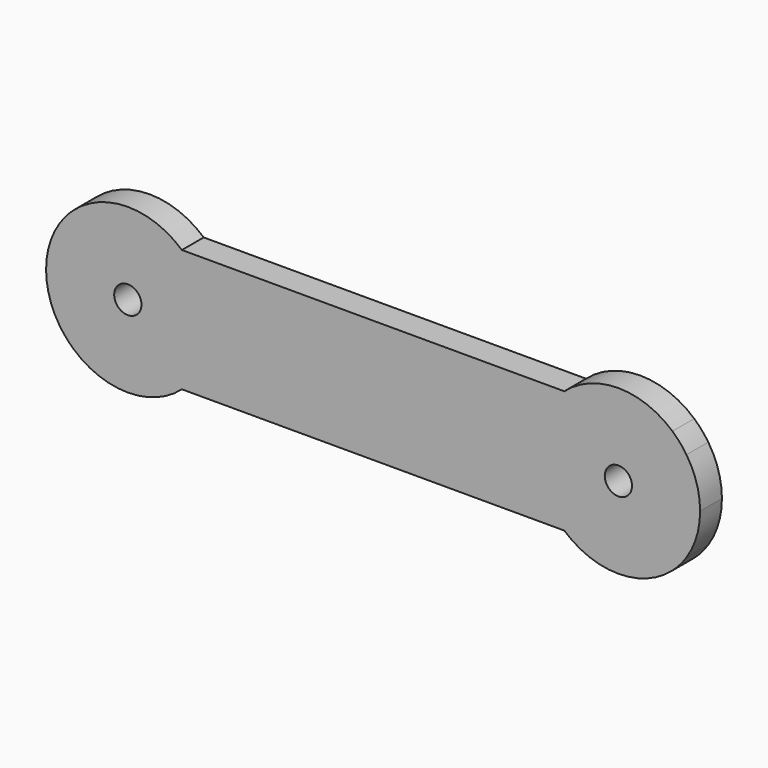
from build123d import *

# Parameters (mm, degrees)
F0_R     = 1
F1_DEPTH = 2


with BuildPart() as f1:
    # F0 (on Front) → F1 (new body)
    with BuildSketch(Plane.XZ):
        with BuildLine():
            ThreePointArc((-49.9391267766, 34.7456367077), (-53.9077537432, 36.2456367077), (-57.8763807098, 34.7456367077))
            Line((-57.8763807098, 34.7456367077), (-49.9391267766, 34.7456367077))
        make_face()
        with BuildLine():
            Line((-49.9391267766, 34.7456367077), (-57.8763807098, 34.7456367077))
            ThreePointArc((-57.8763807098, 34.7456367077), (-58.4309342214, 34.1878237101), (-58.9077537432, 33.562261498))
            Line((-58.9077537432, 33.562261498), (-58.9077537432, 26.9290119173))
            ThreePointArc((-58.9077537432, 26.9290119173), (-58.4309342214, 26.3034497053), (-57.8763807098, 25.7456367077))
            Line((-57.8763807098, 25.7456367077), (-49.9391267766, 25.7456367077))
            ThreePointArc((-49.9391267766, 25.7456367077), (-49.3845732651, 26.3034497053), (-48.9077537432, 26.9290119173))
            Line((-48.9077537432, 26.9290119173), (-48.9077537432, 30.2456367077))
            Line((-48.9077537432, 30.2456367077), (-48.9077537432, 33.562261498))
            ThreePointArc((-48.9077537432, 33.562261498), (-49.3845732651, 34.1878237101), (-49.9391267766, 34.7456367077))
        make_face()
        with Locations((-53.9077537432, 30.2456367077)):
            Circle(F0_R, mode=Mode.SUBTRACT)
        with BuildLine():
            Line((-58.9077537432, 26.9290119173), (-58.9077537432, 33.562261498))
            ThreePointArc((-58.9077537432, 33.562261498), (-59.9077537432, 30.2456367077), (-58.9077537432, 26.9290119173))
        make_face()
        with BuildLine():
            Line((-48.9077537432, 34.7456367077), (-49.9391267766, 34.7456367077))
            ThreePointArc((-49.9391267766, 34.7456367077), (-49.3845732651, 34.1878237101), (-48.9077537432, 33.562261498))
            Line((-48.9077537432, 33.562261498), (-48.9077537432, 34.7456367077))
        make_face()
        with BuildLine():
            Line((-22.9077537432, 34.7456367077), (-48.9077537432, 34.7456367077))
            Line((-48.9077537432, 34.7456367077), (-48.9077537432, 33.562261498))
            ThreePointArc((-48.9077537432, 33.562261498), (-48.1631910967, 31.9776875152), (-47.9077537432, 30.2456367077))
            ThreePointArc((-47.9077537432, 30.2456367077), (-48.1631910967, 28.5135859001), (-48.9077537432, 26.9290119173))
            Line((-48.9077537432, 26.9290119173), (-48.9077537432, 25.7456367077))
            Line((-48.9077537432, 25.7456367077), (-22.9077537432, 25.7456367077))
            Line((-22.9077537432, 25.7456367077), (-22.9077537432, 26.9290119173))
            ThreePointArc((-22.9077537432, 26.9290119173), (-23.9077537432, 30.2456367077), (-22.9077537432, 33.562261498))
            Line((-22.9077537432, 33.562261498), (-22.9077537432, 34.7456367077))
        make_face()
        with BuildLine():
            ThreePointArc((-47.9077537432, 30.2456367077), (-48.1631910967, 31.9776875152), (-48.9077537432, 33.562261498))
            Line((-48.9077537432, 33.562261498), (-48.9077537432, 30.2456367077))
            Line((-48.9077537432, 30.2456367077), (-48.9077537432, 26.9290119173))
            ThreePointArc((-48.9077537432, 26.9290119173), (-48.1631910967, 28.5135859001), (-47.9077537432, 30.2456367077))
        make_face()
        with BuildLine():
            Line((-49.9391267766, 25.7456367077), (-57.8763807098, 25.7456367077))
            ThreePointArc((-57.8763807098, 25.7456367077), (-53.9077537432, 24.2456367077), (-49.9391267766, 25.7456367077))
        make_face()
        with BuildLine():
            Line((-21.8763807098, 34.7456367077), (-22.9077537432, 34.7456367077))
            Line((-22.9077537432, 34.7456367077), (-22.9077537432, 33.562261498))
            ThreePointArc((-22.9077537432, 33.562261498), (-22.4309342214, 34.1878237101), (-21.8763807098, 34.7456367077))
        make_face()
        with BuildLine():
            ThreePointArc((-48.9077537432, 26.9290119173), (-49.3845732651, 26.3034497053), (-49.9391267766, 25.7456367077))
            Line((-49.9391267766, 25.7456367077), (-48.9077537432, 25.7456367077))
            Line((-48.9077537432, 25.7456367077), (-48.9077537432, 26.9290119173))
        make_face()
        with BuildLine():
            ThreePointArc((-13.9391267766, 34.7456367077), (-17.9077537432, 36.2456367077), (-21.8763807098, 34.7456367077))
            Line((-21.8763807098, 34.7456367077), (-13.9391267766, 34.7456367077))
        make_face()
        with BuildLine():
            Line((-13.9391267766, 34.7456367077), (-21.8763807098, 34.7456367077))
            ThreePointArc((-21.8763807098, 34.7456367077), (-22.4309342214, 34.1878237101), (-22.9077537432, 33.562261498))
            Line((-22.9077537432, 33.562261498), (-22.9077537432, 30.2456367077))
            Line((-22.9077537432, 30.2456367077), (-22.9077537432, 26.9290119173))
            ThreePointArc((-22.9077537432, 26.9290119173), (-22.4309342214, 26.3034497053), (-21.8763807098, 25.7456367077))
            Line((-21.8763807098, 25.7456367077), (-13.9391267766, 25.7456367077))
            ThreePointArc((-13.9391267766, 25.7456367077), (-13.3845732651, 26.3034497053), (-12.9077537432, 26.9290119173))
            Line((-12.9077537432, 26.9290119173), (-12.9077537432, 33.562261498))
            ThreePointArc((-12.9077537432, 33.562261498), (-13.3845732651, 34.1878237101), (-13.9391267766, 34.7456367077))
        make_face()
        with BuildLine():
            ThreePointArc((-16.9077537432, 30.2456367077), (-17.9077537432, 29.2456367077), (-18.9077537432, 30.2456367077))
            ThreePointArc((-18.9077537432, 30.2456367077), (-17.9077537432, 31.2456367077), (-16.9077537432, 30.2456367077))
        make_face(mode=Mode.SUBTRACT)
        with BuildLine():
            Line((-22.9077537432, 30.2456367077), (-22.9077537432, 33.562261498))
            ThreePointArc((-22.9077537432, 33.562261498), (-23.9077537432, 30.2456367077), (-22.9077537432, 26.9290119173))
            Line((-22.9077537432, 26.9290119173), (-22.9077537432, 30.2456367077))
        make_face()
        with BuildLine():
            ThreePointArc((-21.8763807098, 25.7456367077), (-22.4309342214, 26.3034497053), (-22.9077537432, 26.9290119173))
            Line((-22.9077537432, 26.9290119173), (-22.9077537432, 25.7456367077))
            Line((-22.9077537432, 25.7456367077), (-21.8763807098, 25.7456367077))
        make_face()
        with BuildLine():
            ThreePointArc((-11.9077537432, 30.2456367077), (-12.1631910967, 31.9776875152), (-12.9077537432, 33.562261498))
            Line((-12.9077537432, 33.562261498), (-12.9077537432, 26.9290119173))
            ThreePointArc((-12.9077537432, 26.9290119173), (-12.1631910967, 28.5135859001), (-11.9077537432, 30.2456367077))
        make_face()
        with BuildLine():
            Line((-13.9391267766, 25.7456367077), (-21.8763807098, 25.7456367077))
            ThreePointArc((-21.8763807098, 25.7456367077), (-17.9077537432, 24.2456367077), (-13.9391267766, 25.7456367077))
        make_face()
    extrude(amount=F1_DEPTH)


solid = f1.part
